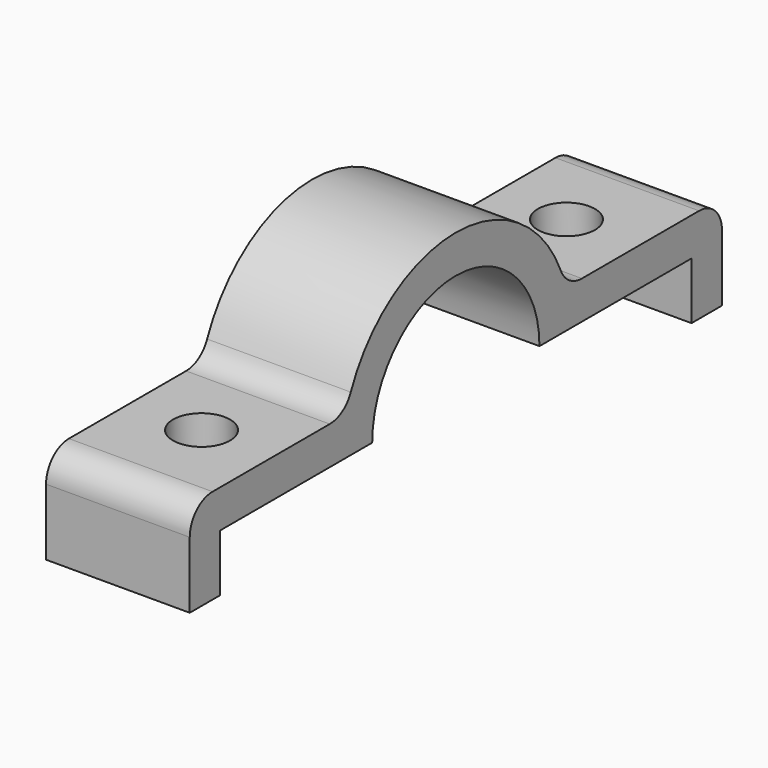
from build123d import *

# Parameters (mm, degrees)
F1_DEPTH  = 24
F2_W      = 48
F2_H      = 12.7
F2_H_2    = 19.05
F3_DEPTH  = 12.7
F4_R      = 9.525
F6_R      = 9.525
F8_DEPTH  = 47.498
F10_DEPTH = 25.4
F5_W      = 48
F5_H      = 19.05
F5_H_2    = 12.7
F11_DEPTH = 12.7
F12_R     = 9.525
F15_DEPTH = 25.4


# Not quite as in the source:
# - two fillets or chamfers of one size are made in one step
# - a feature names something its author has since deleted; it is built from what else it names


with BuildPart() as f1:
    # F0 (on Right) → F1 (new body, symmetric)
    with BuildSketch(Plane.YZ):
        with BuildLine():
            ThreePointArc((-34.925, 0), (0, 34.925), (34.925, 0))
            Line((34.925, 0), (98.425, 0))
            Line((98.425, 0), (98.425, 12.7))
            Line((98.425, 12.7), (87.425, 12.7))
            Line((87.425, 12.7), (45.900442536, 12.7))
            ThreePointArc((45.900442536, 12.7), (0, 47.625), (-45.900442536, 12.7))
            Line((-45.900442536, 12.7), (-98.425, 12.7))
            Line((-98.425, 12.7), (-98.425, 0))
            Line((-98.425, 0), (-34.925, 0))
        make_face()
    extrude(amount=F1_DEPTH, both=True)

    # F2 (on face) → F3 (join)
    with BuildSketch(Plane.XZ.offset(98.425)):
        with Locations((0, 6.35)):
            Rectangle(F2_W, F2_H)
        with Locations((0, -9.525)):
            Rectangle(F2_W, F2_H_2)
    extrude(amount=F3_DEPTH)

    # F4
    f4_edges = [f1.edges().sort_by_distance(p)[0] for p in [
        (0, -111.125, 12.7),
    ]]
    fillet(f4_edges, radius=F4_R)

    # F6
    f6_edges = [f1.edges().sort_by_distance(p)[0] for p in [
        (0, -45.900443, 12.7),
        (0, 45.900443, 12.7),
    ]]
    fillet(f6_edges, radius=F6_R)

    # F7 (on face) → F8 (cut)
    with BuildSketch(Plane(origin=(0, 0, 0), x_dir=(1, 0, 0), z_dir=(0, 0, -1))):
        with BuildLine():
            ThreePointArc((9.525, 76.2), (-6.7351920908, 82.9351920908), (0, 66.675))
            ThreePointArc((0, 66.675), (6.7351920908, 69.4648079092), (9.525, 76.2))
        make_face()
    extrude(amount=-F8_DEPTH, mode=Mode.SUBTRACT)

    # F9 (on face) → F10 (cut)
    with BuildSketch(Plane(origin=(0, 0, 0), x_dir=(1, 0, 0), z_dir=(0, 0, -1))):
        with BuildLine():
            ThreePointArc((9.525, -6.35), (6.7351920908, 0.3851920908), (0, 3.175))
            ThreePointArc((0, 3.175), (-6.7351920908, -13.0851920908), (9.525, -6.35))
        make_face()
    extrude(amount=-F10_DEPTH, mode=Mode.SUBTRACT)

    # F5 (on face) → F11 (join)
    with BuildSketch(Plane(origin=(0, 98.425, 0), x_dir=(-1, 0, 0), z_dir=(0, 1, 0))):
        with Locations((0, -9.525)):
            Rectangle(F5_W, F5_H)
        with Locations((0, 6.35)):
            Rectangle(F5_W, F5_H_2)
    extrude(amount=F11_DEPTH)

    # F12
    f12_edges = [f1.edges().sort_by_distance(p)[0] for p in [
        (0, 111.125, 12.7),
    ]]
    fillet(f12_edges, radius=F12_R)

    # F14 (on face) → F15 (cut)
    with BuildSketch(Plane(origin=(0, 0, 0), x_dir=(1, 0, 0), z_dir=(0, 0, -1))):
        with BuildLine():
            ThreePointArc((9.525, -76.2), (6.7351920908, -69.4648079092), (0, -66.675))
            ThreePointArc((0, -66.675), (-6.7351920908, -82.9351920908), (9.525, -76.2))
        make_face()
    extrude(amount=-F15_DEPTH, mode=Mode.SUBTRACT)


solid = f1.part
